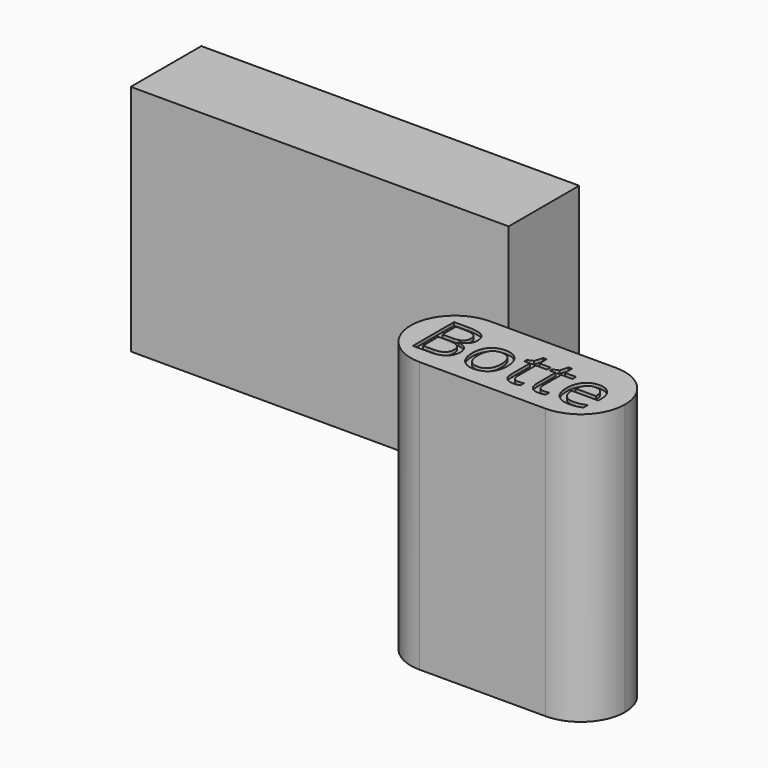
from build123d import *

# Parameters (mm, degrees)
F0_W         = 340
F0_H         = 140
F1_DEPTH     = 430
F2_TEXT_SIZE = 114.5537587952
F3_DEPTH     = 5
F4_R         = 69.99999
F5_W         = 600
F5_H         = 140
F6_DEPTH     = 370
F7_TEXT_SIZE = 101.2973064639
F8_DEPTH     = 5
F9_TEXT_SIZE = 69.5610168468
F10_DEPTH    = 5


# Not quite as in the source:
# - a fillet or chamfer is up to 0.001 mm smaller than in the source, because OpenCascade refuses the exact size
# - Text() gives the source's letters only with a copy of the font that has no kerning and outlines rounded to 1/6400 em; it was checked with that copy


with BuildPart() as f1:
    # F0 (on Top) → F1 (new body)
    with BuildSketch(Plane.XY):
        Rectangle(F0_W, F0_H)
    extrude(amount=F1_DEPTH)

    # F2 (on face) → F3 (cut)
    with BuildSketch(Plane.XY.offset(430)):
        with Locations((-145, -41.2393531663)):
            Text('Botte', F2_TEXT_SIZE, font='Open Sans', text_align=(TextAlign.LEFT, TextAlign.BOTTOM))
    extrude(amount=-F3_DEPTH, mode=Mode.SUBTRACT)

    # F4 (radius 70 in the source; OpenCascade refuses exactly that, so slightly less here)
    f4_edges = [f1.edges().sort_by_distance(p)[0] for p in [
        (-170, -70, 215),
        (-170, 70, 215),
        (170, -70, 215),
        (170, 70, 215),
    ]]
    fillet(f4_edges, radius=F4_R)


with BuildPart() as f6:
    # F5 (on Top) → F6 (new body)
    with BuildSketch(Plane.XY):
        with Locations((-613.3684337139, 443.4096288681)):
            Rectangle(F5_W, F5_H)
    extrude(amount=F6_DEPTH)

    # F7 (on face) → F8 (cut)
    with BuildSketch(Plane(origin=(0, 513.4096288681, 0), x_dir=(-1, 0, 0), z_dir=(0, 1, 0))):
        with Locations((333.3684337139, 148.532969673)):
            Text('Boitte botte', F7_TEXT_SIZE, font='Open Sans', text_align=(TextAlign.LEFT, TextAlign.BOTTOM))
    extrude(amount=-F8_DEPTH, mode=Mode.SUBTRACT)

    # F9 (on face) → F10 (cut)
    with BuildSketch(Plane(origin=(-913.3684337139, 0, 0), x_dir=(0, -1, 0), z_dir=(-1, 0, 0))):
        with Locations(Location((-468.451594933, 365), (0, 0, -90))):
            Text('Boite botte', F9_TEXT_SIZE, font='Open Sans', text_align=(TextAlign.LEFT, TextAlign.BOTTOM))
    extrude(amount=-F10_DEPTH, mode=Mode.SUBTRACT)


solid = Compound([f1.part, f6.part])
